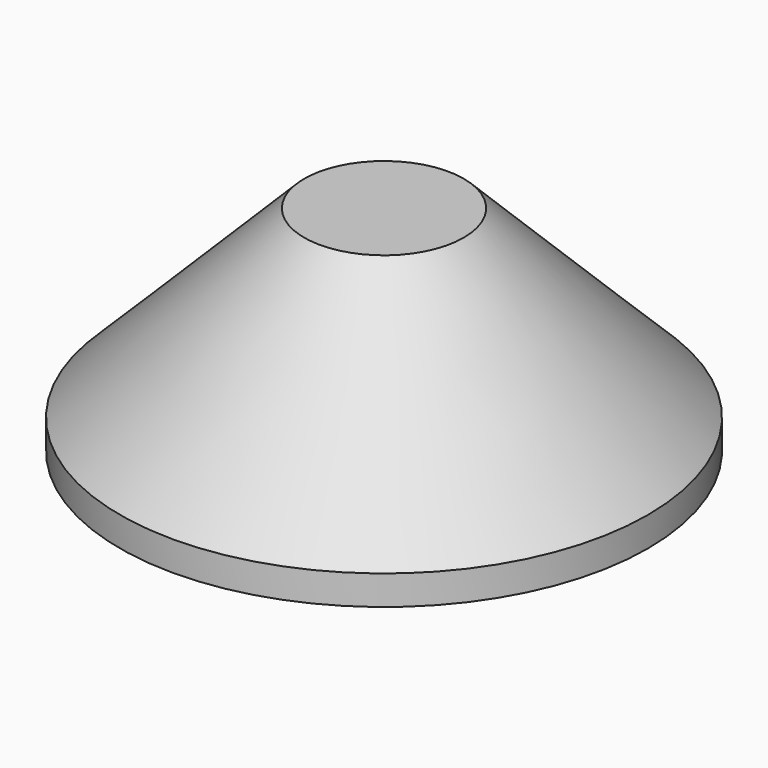
from build123d import *

# Parameters (mm, degrees)
F0_R     = 32.7640800534
F1_DEPTH = 38.1
F2_SIZE  = 22.86
F3_SIZE  = 5.08


# Not quite as in the source:
# - a fillet or chamfer that OpenCascade refuses, or shapes differently, is made with other operations: its cross-section is extruded or revolved along the edge and cut away or added


with BuildPart() as f1:
    # F0 (on Top) → F1 (new body)
    with BuildSketch(Plane.XY):
        Circle(F0_R)
    extrude(amount=F1_DEPTH)

    # F2
    f2_edges = [f1.edges().sort_by_distance(p)[0] for p in [
        (-32.76408, 0, 38.1),
    ]]
    chamfer(f2_edges, length=F2_SIZE)

    # F3
    f3_edges = [f1.edges().sort_by_distance(p)[0] for p in [
        (-32.76408, 0, 0),
    ]]
    chamfer(f3_edges, length=F3_SIZE)

    # F4: chamfer of 22.86 on 1 edges, made by hand

    # F4_s1 → F4_t2 (revolve, cut)
    with BuildSketch(Plane.XZ):
        Polygon((43.8485410713, 16.1644610179), (4.8240800534, 0), (27.6840800534, 0), align=None)
    revolve(axis=Axis((0, 0, 0), (0, 0, 1)), mode=Mode.SUBTRACT)


solid = f1.part
